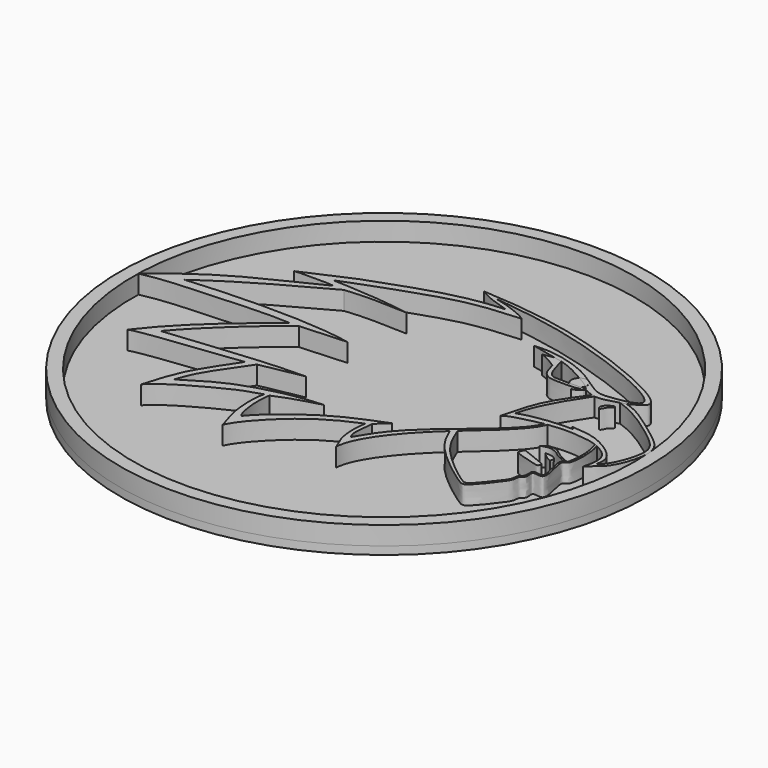
from build123d import *

# Parameters (mm, degrees)
F0_R     = 20
F1_DEPTH = 0.6
F2_R     = 20
F2_R_2   = 19
F3_DEPTH = 1.4
F5_DEPTH = 1.4
F6_DEPTH = 1.4


with BuildPart() as f1:
    # F0 (on Top) → F1 (new body)
    with BuildSketch(Plane.XY):
        Circle(F0_R)
    extrude(amount=-F1_DEPTH)

    # F2 (on Top) → F3 (join)
    with BuildSketch(Plane.XY):
        Circle(F2_R)
        Circle(F2_R_2, mode=Mode.SUBTRACT)
    extrude(amount=F3_DEPTH)


with BuildPart() as f5:
    # F4 (on Top) → F5 (new body)
    with BuildSketch(Plane.XY):
        with BuildLine():
            add(Edge.make_bspline(
                [(-0.4861813504, 11.1744105816), (-0.8512394251, 11.2638310445), (-1.2162974998, 11.3714220446), (-1.5813555744, 11.4608425075)],
                knots=[0, 0, 0, 0, 1.1320114085, 1.1320114085, 1.1320114085, 1.1320114085], degree=3))
            add(Edge.make_bspline(
                [(0.8560517081, 10.4608425075), (0.4573200056, 10.5881941765), (-0.7648135611, 10.9467365684), (-1.4453119288, 11.3807328225), (-1.5813555744, 11.4608425075)],
                knots=[0, 0, 0, 0, 0.579016689, 1, 1, 1, 1], degree=3))
            add(Edge.make_bspline(
                [(0.8560517081, 10.4608425075), (1.347997395, 10.3502387475), (1.8399430819, 10.2214644504), (2.3318887688, 10.1108606905)],
                knots=[0, 0, 0, 0, 1.5167670559, 1.5167670559, 1.5167670559, 1.5167670559], degree=3))
            add(Edge.make_bspline(
                [(-0.4861813504, 11.1744105816), (-0.0018532867, 11.0755696507), (0.8729949517, 10.8262661766), (2.0316981245, 10.3485118598), (2.3318887688, 10.1108606905)],
                knots=[0, 0, 0, 0, 0.493621531, 1, 1, 1, 1], degree=3))
        make_face()
        with BuildLine():
            add(Edge.make_bspline(
                [(-1.5813555744, 11.4608425075), (1.514651197, 11.2793503488), (6.8334553558, 10.6998128091), (16.2828207566, 6.5822660882), (14.74853224, 5.8477105562), (14.0055896595, 5.4608425075)],
                knots=[0, 0, 0, 0, 0.4316285007, 0.8324272833, 1, 1, 1, 1], degree=3))
            add(Edge.make_bspline(
                [(-0.4861813504, 11.1744105816), (-0.8512394251, 11.2638310445), (-1.2162974998, 11.3714220446), (-1.5813555744, 11.4608425075)],
                knots=[0, 0, 0, 0, 1.1320114085, 1.1320114085, 1.1320114085, 1.1320114085], degree=3))
            add(Edge.make_bspline(
                [(10.5331156468, 6.2760727313), (10.9363930891, 6.0023009623), (11.7608523883, 5.4283523122), (12.6827028969, 5.4977681276), (16.7129876566, 6.1384112415), (6.8471463505, 10.2922851198), (1.9949780392, 10.875952097), (-0.4861813504, 11.1744105816)],
                knots=[0.2889714832, 0.2889714832, 0.2889714832, 0.2889714832, 0.356550035, 0.445023231, 0.5537782213, 0.7718242062, 1, 1, 1, 1], degree=3))
            ThreePointArc((10.5331156468, 6.2760727313), (10.5980424704, 6.205178512), (10.6508136936, 6.1248250382))
            add(Edge.make_bspline(
                [(10.6738684154, 6.0779841061), (10.6672489525, 6.0941943415), (10.6595052577, 6.109775343), (10.6508136936, 6.1248250382)],
                knots=[0.5200267079, 0.5200267079, 0.5200267079, 0.5200267079, 0.5950226776, 0.5950226776, 0.5950226776, 0.5950226776], degree=3))
            ThreePointArc((10.6738684154, 6.0779841061), (10.7117232873, 5.9599696048), (10.7245236322, 5.8366952562))
            ThreePointArc((10.7245236322, 5.8366952562), (10.7193245726, 5.7578800215), (10.7038174948, 5.6804306704))
            add(Edge.make_bspline(
                [(10.8788917387, 5.514291408), (10.8202111372, 5.5743074932), (10.7620872809, 5.6292667311), (10.7038174948, 5.6804306704)],
                knots=[0.0457537508, 0.0457537508, 0.0457537508, 0.0457537508, 0.1098862637, 0.1098862637, 0.1098862637, 0.1098862637], degree=3))
            add(Edge.make_bspline(
                [(11.0055896595, 5.3776609224), (10.9629035479, 5.4260836214), (10.9207559585, 5.4714744204), (10.8788917387, 5.514291408)],
                knots=[0, 0, 0, 0, 0.0457537508, 0.0457537508, 0.0457537508, 0.0457537508], degree=3))
            add(Edge.make_bspline(
                [(11.7051415145, 5.0738393329), (11.478102131, 5.1392894421), (11.2418546361, 5.258068017), (11.0055896595, 5.3776609224)],
                knots=[0.7087711743, 0.7087711743, 0.7087711743, 0.7087711743, 1, 1, 1, 1], degree=3))
            add(Edge.make_bspline(
                [(11.9165486953, 5.0284702119), (11.8452559027, 5.038333895), (11.7756426549, 5.0535155139), (11.7051415145, 5.0738393329)],
                knots=[0.6183376821, 0.6183376821, 0.6183376821, 0.6183376821, 0.7087711743, 0.7087711743, 0.7087711743, 0.7087711743], degree=3))
            add(Edge.make_bspline(
                [(13.5997429191, 5.3412596545), (13.1580057928, 5.2100697092), (12.4957655955, 5.0153138893), (12.0665301911, 5.0077195875), (11.9165486953, 5.0284702119)],
                knots=[0.0995715401, 0.0995715401, 0.0995715401, 0.0995715401, 0.4280891318, 0.6183376821, 0.6183376821, 0.6183376821, 0.6183376821], degree=3))
            add(Edge.make_bspline(
                [(14.0055896595, 5.4608425075), (13.8695725155, 5.4215071201), (13.7336305619, 5.3810224715), (13.5997429191, 5.3412596545)],
                knots=[0, 0, 0, 0, 0.0995715401, 0.0995715401, 0.0995715401, 0.0995715401], degree=3))
        make_face()
        with BuildLine():
            add(Edge.make_bspline(
                [(0.8560517081, 10.4608425075), (1.347997395, 10.3502387475), (1.8399430819, 10.2214644504), (2.3318887688, 10.1108606905)],
                knots=[0, 0, 0, 0, 1.5167670559, 1.5167670559, 1.5167670559, 1.5167670559], degree=3))
            add(Edge.make_bspline(
                [(-11.9944103405, 6.4608425075), (-7.4352765712, 8.5330202898), (-8.3438375258, 7.8825665939), (-2.5707737153, 10.3058462526), (0.8560517081, 10.4608425075)],
                knots=[0, 0, 0, 0, 0.454663222, 1, 1, 1, 1], degree=3))
            add(Edge.make_bspline(
                [(-9.437805973, 6.9979857653), (-10.2901514814, 6.812881167), (-11.1420648321, 6.6459471058), (-11.9944103405, 6.4608425075)],
                knots=[0, 0, 0, 0, 2.6124220125, 2.6124220125, 2.6124220125, 2.6124220125], degree=3))
            add(Edge.make_bspline(
                [(2.3318887688, 10.1108606905), (-0.1704881142, 9.9523263052), (-2.4060494059, 9.6797784859), (-8.1382575205, 7.5277293123), (-9.437805973, 6.9979857653)],
                knots=[0, 0, 0, 0, 0.4735027483, 1, 1, 1, 1], degree=3))
        make_face()
        with BuildLine():
            add(Edge.make_bspline(
                [(-9.437805973, 6.9979857653), (-10.2901514814, 6.812881167), (-11.1420648321, 6.6459471058), (-11.9944103405, 6.4608425075)],
                knots=[0, 0, 0, 0, 2.6124220125, 2.6124220125, 2.6124220125, 2.6124220125], degree=3))
            add(Edge.make_bspline(
                [(-8.9944103405, 6.4608425075), (-9.5227345876, 6.5312589572), (-10.5059407944, 6.462516723), (-11.5227462601, 6.5312941655), (-11.9944103405, 6.4608425075)],
                knots=[0, 0, 0, 0, 0.5049792134, 1, 1, 1, 1], degree=3))
            add(Edge.make_bspline(
                [(-8.9944103405, 6.4608425075), (-8.6776053034, 6.6301364597), (-8.397439304, 6.7902582409), (-8.1671202768, 6.9393072683)],
                knots=[0.8832644452, 0.8832644452, 0.8832644452, 0.8832644452, 0.9755031654, 0.9755031654, 0.9755031654, 0.9755031654], degree=3))
            add(Edge.make_bspline(
                [(-9.437805973, 6.9979857653), (-9.0126793763, 6.9801507696), (-8.5877041172, 6.9611772663), (-8.1671202768, 6.9393072683)],
                knots=[0, 0, 0, 0, 0.199815969, 0.199815969, 0.199815969, 0.199815969], degree=3))
        make_face()
        with BuildLine():
            add(Edge.make_bspline(
                [(8.0055896595, -3.7900607299), (8.290317767, -4.4521385807), (8.9844809049, -5.9540217767), (12.3723434925, -8.4515768964), (13.0451164666, -8.7486977353), (14.3514148065, -7.0178963679), (14.8895121762, -6.3201394359), (14.8316541913, -5.6999676159), (15.339054605, -5.5833601899), (14.9418951503, -4.6397911415), (16.5155754804, -5.3697956819), (15.4397338992, -2.7507088417), (15.9484677785, -2.6639513417), (16.2027573046, -2.339614399), (16.3157848864, -0.8692982274), (16.0055896595, 0.1406914093)],
                knots=[0, 0, 0, 0, 0.1137784461, 0.2601902701, 0.3148507936, 0.417422291, 0.4884856376, 0.539189381, 0.5832073247, 0.6383062782, 0.7002794606, 0.8033644458, 0.8434914934, 0.8846524249, 1, 1, 1, 1], degree=3))
            add(Edge.make_bspline(
                [(16.0055896595, 0.1406914093), (15.936859435, 0.1718639514), (15.8688960906, 0.2002961396), (15.8029496035, 0.2260058139)],
                knots=[0.4452740587, 0.4452740587, 0.4452740587, 0.4452740587, 0.4779418896, 0.4779418896, 0.4779418896, 0.4779418896], degree=3))
            add(Edge.make_bspline(
                [(15.8029496035, 0.2260058139), (16.2006936994, -0.9693456093), (15.9668899378, -2.2166192794), (15.92795558, -2.5949034419), (15.2159733402, -2.5941041989), (16.3932154949, -5.2814039939), (14.8734115826, -4.438489823), (15.1842299283, -5.5488731457), (14.6978233661, -5.6306795332), (14.7380276879, -6.2892111084), (14.2456086984, -6.8848450801), (13.0376296594, -8.4664264452), (12.4637437687, -8.3038412893), (9.1357052886, -5.7276571911), (8.6434670243, -4.1571202739), (8.3486537341, -3.4801096134)],
                knots=[0, 0, 0, 0, 0.1170783241, 0.1538590408, 0.1984892764, 0.3021938664, 0.3631383845, 0.4243811494, 0.4678027754, 0.5205636841, 0.5883717685, 0.6881215272, 0.7381813319, 0.8845935619, 1, 1, 1, 1], degree=3))
            add(Edge.make_bspline(
                [(8.0055896595, -3.7900607299), (8.1183412502, -3.6872860039), (8.2326324706, -3.5841350133), (8.3486537341, -3.4801096134)],
                knots=[0.5563520178, 0.5563520178, 0.5563520178, 0.5563520178, 0.5913081958, 0.5913081958, 0.5913081958, 0.5913081958], degree=3))
        make_face()
        with BuildLine():
            add(Edge.make_bspline(
                [(-8.9944103405, 6.4608425075), (-8.7216751352, 6.456489241), (-8.4493720874, 6.4339654374), (-8.1766368821, 6.4296121709)],
                knots=[0, 0, 0, 0, 0.8183695761, 0.8183695761, 0.8183695761, 0.8183695761], degree=3))
            add(Edge.make_bspline(
                [(-18.9944103405, 0.4608425075), (-17.5819190405, 1.6336166373), (-14.9380365277, 3.719038189), (-10.3751922712, 5.7229816691), (-8.9944103405, 6.4608425075)],
                knots=[0, 0, 0, 0, 0.4812457167, 0.8832644452, 0.8832644452, 0.8832644452, 0.8832644452], degree=3))
            add(Edge.make_bspline(
                [(-16.3652878255, 1.5516962158), (-17.2418060497, 1.1820214673), (-18.1178921163, 0.8305172559), (-18.9944103405, 0.4608425075)],
                knots=[0, 0, 0, 0, 2.8464446265, 2.8464446265, 2.8464446265, 2.8464446265], degree=3))
            add(Edge.make_bspline(
                [(-8.1766368821, 6.4296121709), (-10.0553413983, 5.4250495729), (-13.461796709, 3.559962101), (-15.4947216945, 2.1565062864), (-16.3652878255, 1.5516962158)],
                knots=[0, 0, 0, 0, 0.571381465, 1, 1, 1, 1], degree=3))
        make_face()
        with BuildLine():
            add(Edge.make_bspline(
                [(-8.9944103405, 6.4608425075), (-8.6776053034, 6.6301364597), (-8.397439304, 6.7902582409), (-8.1671202768, 6.9393072683)],
                knots=[0.8832644452, 0.8832644452, 0.8832644452, 0.8832644452, 0.9755031654, 0.9755031654, 0.9755031654, 0.9755031654], degree=3))
            add(Edge.make_bspline(
                [(-8.9944103405, 6.4608425075), (-8.7216751352, 6.456489241), (-8.4493720874, 6.4339654374), (-8.1766368821, 6.4296121709)],
                knots=[0, 0, 0, 0, 0.8183695761, 0.8183695761, 0.8183695761, 0.8183695761], degree=3))
            add(Edge.make_bspline(
                [(-3.4766462632, 6.4608425075), (-4.6195223532, 6.4761082239), (-6.0056012046, 6.5942768078), (-7.709692655, 6.4793701805), (-8.1766368821, 6.4296121709)],
                knots=[0, 0, 0, 0, 0.5412673538, 1, 1, 1, 1], degree=3))
            add(Edge.make_bspline(
                [(-8.1671202768, 6.9393072683), (-7.4883861721, 6.9040136786), (-5.8324939664, 6.79771411), (-4.3567601819, 6.5994669238), (-3.4766462632, 6.4608425075)],
                knots=[0.199815969, 0.199815969, 0.199815969, 0.199815969, 0.5222770334, 1, 1, 1, 1], degree=3))
        make_face()
        with BuildLine():
            add(Edge.make_bspline(
                [(4.0055896595, -9.5391574925), (4.0640229048, -8.4050470974), (5.6258918331, -6.0675921748), (7.2579217171, -4.4715710079), (8.0055896595, -3.7900607299)],
                knots=[0, 0, 0, 0, 0.3245538369, 0.5563520178, 0.5563520178, 0.5563520178, 0.5563520178], degree=3))
            add(Edge.make_bspline(
                [(8.0055896595, -3.7900607299), (8.1183412502, -3.6872860039), (8.2326324706, -3.5841350133), (8.3486537341, -3.4801096134)],
                knots=[0.5563520178, 0.5563520178, 0.5563520178, 0.5563520178, 0.5913081958, 0.5913081958, 0.5913081958, 0.5913081958], degree=3))
            add(Edge.make_bspline(
                [(8.3486537341, -3.4801096134), (8.5877905191, -3.2656980569), (9.9859491551, -2.0284086781), (11.6742389457, -0.5312455851), (12.0055896595, 0.4608425075)],
                knots=[0.5913081958, 0.5913081958, 0.5913081958, 0.5913081958, 0.6633579887, 1, 1, 1, 1], degree=3))
            add(Edge.make_bspline(
                [(11.8052601549, 0.4324009459), (11.8704997149, 0.4414805342), (11.9403500995, 0.4517629192), (12.0055896595, 0.4608425075)],
                knots=[0, 0, 0, 0, 0.2023384117, 0.2023384117, 0.2023384117, 0.2023384117], degree=3))
            add(Edge.make_bspline(
                [(3.9102742448, -8.0432752147), (4.3585507686, -7.225709157), (5.503324856, -5.5090435402), (8.5702876807, -2.9413221208), (11.3297734442, -0.6915840851), (11.8052601549, 0.4324009459)],
                knots=[0, 0, 0, 0, 0.2886820024, 0.6363748963, 1, 1, 1, 1], degree=3))
            add(Edge.make_bspline(
                [(3.8548011798, -5.9568551369), (3.772172657, -6.5835202766), (3.644234835, -7.5538168559), (3.8406969894, -7.9152672279), (3.9102742448, -8.0432752147)],
                knots=[0, 0, 0, 0, 0.6458490662, 1, 1, 1, 1], degree=3))
            add(Edge.make_bspline(
                [(3.5055896595, -6.1596883461), (3.6221375521, -6.0920772764), (3.7382532872, -6.0244662066), (3.8548011798, -5.9568551369)],
                knots=[0, 0, 0, 0, 0.4038440252, 0.4038440252, 0.4038440252, 0.4038440252], degree=3))
            add(Edge.make_bspline(
                [(3.5055896595, -6.1596883461), (3.3600590635, -6.9084815459), (3.4432477493, -8.5297381785), (3.7729906459, -8.9020562877), (4.0055896595, -9.5391574925)],
                knots=[0, 0, 0, 0, 0.5658292742, 1, 1, 1, 1], degree=3))
        make_face()
        with BuildLine():
            add(Edge.make_bspline(
                [(-16.3652878255, 1.5516962158), (-17.2418060497, 1.1820214673), (-18.1178921163, 0.8305172559), (-18.9944103405, 0.4608425075)],
                knots=[0, 0, 0, 0, 2.8464446265, 2.8464446265, 2.8464446265, 2.8464446265], degree=3))
            add(Edge.make_bspline(
                [(-7.9944103405, 1.1069288947), (-9.4193134786, 1.237536743), (-13.8743454501, 0.9399078326), (-17.3496462389, 0.824787051), (-18.9944103405, 0.4608425075)],
                knots=[0, 0, 0, 0, 0.5087005402, 1, 1, 1, 1], degree=3))
            add(Edge.make_bspline(
                [(-7.9944103405, 1.1069288947), (-7.7784326722, 1.118545444), (-7.5628871615, 1.1301619933), (-7.3469094932, 1.1417785427)],
                knots=[0, 0, 0, 0, 0.6484380041, 0.6484380041, 0.6484380041, 0.6484380041], degree=3))
            add(Edge.make_bspline(
                [(-3.8513934705, 1.3500220375), (-5.0165654781, 1.2806075392), (-6.1817374857, 1.2111930409), (-7.3469094932, 1.1417785427)],
                knots=[0, 0, 0, 0, 3.501713526, 3.501713526, 3.501713526, 3.501713526], degree=3))
            add(Edge.make_bspline(
                [(-16.3652878255, 1.5516962158), (-15.565707993, 1.6230606445), (-13.3888340962, 1.8009877733), (-6.9601712748, 1.95987802), (-3.8513934705, 1.3500220375)],
                knots=[0, 0, 0, 0, 0.3529099079, 1, 1, 1, 1], degree=3))
        make_face()
        with BuildLine():
            add(Edge.make_bspline(
                [(11.8052601549, 0.4324009459), (11.8704997149, 0.4414805342), (11.9403500995, 0.4517629192), (12.0055896595, 0.4608425075)],
                knots=[0, 0, 0, 0, 0.2023384117, 0.2023384117, 0.2023384117, 0.2023384117], degree=3))
            add(Edge.make_bspline(
                [(12.0055896595, 0.4608425075), (11.9332310752, 0.4510848131), (11.8667309035, 0.4416234795), (11.8052601549, 0.4324009459)],
                knots=[0, 0, 0, 0, 0.0453625168, 0.0453625168, 0.0453625168, 0.0453625168], degree=3))
        make_face()
        with BuildLine():
            add(Edge.make_bspline(
                [(11.0055896595, 5.3776609224), (10.9768566842, 5.3499833826), (10.9481051428, 5.3223087447), (10.9193240765, 5.2950871694)],
                knots=[0, 0, 0, 0, 0.1162457919, 0.1162457919, 0.1162457919, 0.1162457919], degree=3))
            add(Edge.make_bspline(
                [(11.0055896595, 5.3776609224), (10.9629035479, 5.4260836214), (10.9207559585, 5.4714744204), (10.8788917387, 5.514291408)],
                knots=[0, 0, 0, 0, 0.0457537508, 0.0457537508, 0.0457537508, 0.0457537508], degree=3))
            add(Edge.make_bspline(
                [(10.7126522699, 5.2433540713), (10.7778732235, 5.3274456432), (10.828419646, 5.4209023466), (10.8788917387, 5.514291408)],
                knots=[0.6310392789, 0.6310392789, 0.6310392789, 0.6310392789, 1, 1, 1, 1], degree=3))
            add(Edge.make_bspline(
                [(10.7126522759, 5.24335406), (10.7999302605, 5.2588050266), (10.8708150905, 5.2773339919), (10.912349001, 5.291994101), (10.9193240765, 5.2950871694)],
                knots=[0.8539309447, 0.8539309447, 0.8539309447, 0.8539309447, 0.9271004176, 0.9428592974, 0.9428592974, 0.9428592974, 0.9428592974], degree=3))
        make_face()
        with BuildLine():
            add(Edge.make_bspline(
                [(-7.9944103405, 1.1069288947), (-7.7784326722, 1.118545444), (-7.5628871615, 1.1301619933), (-7.3469094932, 1.1417785427)],
                knots=[0, 0, 0, 0, 0.6484380041, 0.6484380041, 0.6484380041, 0.6484380041], degree=3))
            add(Edge.make_bspline(
                [(-14.9944103405, -5.5391574925), (-13.7942935133, -3.9556998013), (-11.3643048238, -1.5615426011), (-8.5238665029, 0.7570548369), (-7.9944103405, 1.1069288947)],
                knots=[0, 0, 0, 0, 0.5500986234, 1, 1, 1, 1], degree=3))
            add(Edge.make_bspline(
                [(-13.3645571768, -4.4584060088), (-13.9079856172, -4.8247133491), (-14.4509819001, -5.1728501522), (-14.9944103405, -5.5391574925)],
                knots=[0, 0, 0, 0, 1.9556188547, 1.9556188547, 1.9556188547, 1.9556188547], degree=3))
            add(Edge.make_bspline(
                [(-7.3469094932, 1.1417785427), (-8.4448163694, 0.338849624), (-10.428148874, -1.3877723247), (-12.459579288, -3.3913620914), (-13.3645571768, -4.4584060088)],
                knots=[0, 0, 0, 0, 0.4931522989, 1, 1, 1, 1], degree=3))
        make_face()
        with BuildLine():
            add(Edge.make_bspline(
                [(3.5055896595, -6.1596883461), (1.5482186348, -6.9707707492), (-0.6694731698, -8.506315502), (-2.5806236884, -10.6681760377), (-2.9944103405, -11.5391574925)],
                knots=[0, 0, 0, 0, 0.5459799602, 1, 1, 1, 1], degree=3))
            add(Edge.make_bspline(
                [(3.5055896595, -6.1596883461), (3.6221375521, -6.0920772764), (3.7382532872, -6.0244662066), (3.8548011798, -5.9568551369)],
                knots=[0, 0, 0, 0, 0.4038440252, 0.4038440252, 0.4038440252, 0.4038440252], degree=3))
            add(Edge.make_bspline(
                [(4.7053410672, -5.1438389346), (4.1925152764, -5.5566010997), (4.1383144756, -5.6858497361), (3.8548011798, -5.9568551369)],
                knots=[0, 0, 0, 0, 1.1766109999, 1.1766109999, 1.1766109999, 1.1766109999], degree=3))
            add(Edge.make_bspline(
                [(-2.8363403399, -9.9698845297), (-2.2336716839, -9.1870877606), (0.8173735421, -6.6037034172), (3.4794779633, -5.6316827497), (4.7053410672, -5.1438389346)],
                knots=[0, 0, 0, 0, 0.5101080536, 1, 1, 1, 1], degree=3))
            add(Edge.make_bspline(
                [(-2.8363403399, -9.9698845297), (-2.8891743926, -10.499032363), (-2.9415762878, -11.0100096592), (-2.9944103405, -11.5391574925)],
                knots=[0, 0, 0, 0, 1.5772139224, 1.5772139224, 1.5772139224, 1.5772139224], degree=3))
        make_face()
        with BuildLine():
            add(Edge.make_bspline(
                [(10.7126522699, 5.2433540713), (10.7778732235, 5.3274456432), (10.828419646, 5.4209023466), (10.8788917387, 5.514291408)],
                knots=[0.6310392789, 0.6310392789, 0.6310392789, 0.6310392789, 1, 1, 1, 1], degree=3))
            add(Edge.make_bspline(
                [(10.5876969687, 5.4552893565), (10.7120407688, 5.4688463016), (10.8133734046, 5.4879357632), (10.8788917387, 5.514291408)],
                knots=[0.9288848526, 0.9288848526, 0.9288848526, 0.9288848526, 1, 1, 1, 1], degree=3))
            ThreePointArc((10.5876969687, 5.4552893565), (10.1438280298, 5.2370058864), (9.686839216, 5.4262901493))
            add(Edge.make_bspline(
                [(7.5754439722, 7.3132768172), (7.7364737299, 6.7638616103), (7.9648004439, 5.8004228314), (8.4151602101, 5.4504426739), (8.6409937872, 5.4554326027), (9.3331000431, 5.4294527687), (9.686839216, 5.4262901493)],
                knots=[0, 0, 0, 0, 0.3160564432, 0.4833699083, 0.6372331155, 0.7893674455, 0.7893674455, 0.7893674455, 0.7893674455], degree=3))
            add(Edge.make_bspline(
                [(7.0055896595, 7.4340827679), (7.1942274201, 7.3945596872), (7.3868062116, 7.3527998979), (7.5754439722, 7.3132768172)],
                knots=[0, 0, 0, 0, 0.5825186824, 0.5825186824, 0.5825186824, 0.5825186824], degree=3))
            add(Edge.make_bspline(
                [(7.0055896595, 7.4340827679), (7.2380322538, 7.1423215901), (7.3789222386, 6.8507832218), (7.476943944, 6.5867935747)],
                knots=[0, 0, 0, 0, 0.1155563183, 0.1155563183, 0.1155563183, 0.1155563183], degree=3))
            add(Edge.make_bspline(
                [(7.476943944, 6.5867935747), (7.5999064538, 6.2556339662), (7.7042415865, 5.7146182621), (8.0113414198, 5.4199653425), (8.4127104593, 5.1092583158), (10.1484899112, 5.1607212843), (10.6451011692, 5.2313953753), (10.7126522759, 5.24335406)],
                knots=[0.1155563183, 0.1155563183, 0.1155563183, 0.1155563183, 0.2605149769, 0.3880464278, 0.5226573434, 0.7972994941, 0.8539309447, 0.8539309447, 0.8539309447, 0.8539309447], degree=3))
        make_face()
        with BuildLine():
            add(Edge.make_bspline(
                [(10.9193240765, 5.2950871694), (10.8136287363, 5.1951188902), (10.5939974651, 5.0008170496), (10.370333691, 4.9282497859), (10.2546671405, 4.8907813616)],
                knots=[0.1162457919, 0.1162457919, 0.1162457919, 0.1162457919, 0.5431458381, 1, 1, 1, 1], degree=3))
            add(Edge.make_bspline(
                [(10.7126522759, 5.24335406), (10.7999302605, 5.2588050266), (10.8708150905, 5.2773339919), (10.912349001, 5.291994101), (10.9193240765, 5.2950871694)],
                knots=[0.8539309447, 0.8539309447, 0.8539309447, 0.8539309447, 0.9271004176, 0.9428592974, 0.9428592974, 0.9428592974, 0.9428592974], degree=3))
            add(Edge.make_bspline(
                [(10.2546671405, 4.8907813616), (10.3986650181, 4.9756816362), (10.5737070223, 5.0788817123), (10.6928685377, 5.2178462391), (10.7126522699, 5.2433540713)],
                knots=[0, 0, 0, 0, 0.5191209503, 0.6310392789, 0.6310392789, 0.6310392789, 0.6310392789], degree=3))
        make_face()
        with BuildLine():
            add(Edge.make_bspline(
                [(-13.3645571768, -4.4584060088), (-13.9079856172, -4.8247133491), (-14.4509819001, -5.1728501522), (-14.9944103405, -5.5391574925)],
                knots=[0, 0, 0, 0, 1.9556188547, 1.9556188547, 1.9556188547, 1.9556188547], degree=3))
            add(Edge.make_bspline(
                [(-6.9944103405, -4.4383769855), (-8.0951718683, -4.5501379279), (-8.9273283999, -4.7239324162), (-14.1716016041, -5.2542345674), (-14.9944103405, -5.5391574925)],
                knots=[0, 0, 0, 0, 0.4007344326, 1, 1, 1, 1], degree=3))
            add(Edge.make_bspline(
                [(-6.9944103405, -4.4383769855), (-6.7415432408, -4.3755271472), (-6.4891082987, -4.3126773089), (-6.2362411991, -4.2498274706)],
                knots=[0, 0, 0, 0, 0.7812626745, 0.7812626745, 0.7812626745, 0.7812626745], degree=3))
            add(Edge.make_bspline(
                [(-3.0233417638, -3.6399713717), (-4.0005971612, -3.8386157244), (-5.4580878496, -4.0878689765), (-6.0480198511, -4.2227470447), (-6.2362411991, -4.2498274706)],
                knots=[0, 0, 0, 0, 0.6546808205, 1, 1, 1, 1], degree=3))
            add(Edge.make_bspline(
                [(-13.3645571768, -4.4584060088), (-12.0681423322, -4.3195819823), (-9.1183843322, -4.0484323098), (-5.700757727, -3.6697206087), (-3.0233417638, -3.6399713717)],
                knots=[0, 0, 0, 0, 0.443130057, 1, 1, 1, 1], degree=3))
        make_face()
        with BuildLine():
            add(Edge.make_bspline(
                [(7.0055896595, 7.4340827679), (7.2380322538, 7.1423215901), (7.3789222386, 6.8507832218), (7.476943944, 6.5867935747)],
                knots=[0, 0, 0, 0, 0.1155563183, 0.1155563183, 0.1155563183, 0.1155563183], degree=3))
            add(Edge.make_bspline(
                [(7.0055896595, 7.4340827679), (6.8483246088, 7.4388027019), (6.526745131, 7.363842235), (6.3055163314, 7.3433438763), (6.1365221627, 7.2932951152)],
                knots=[0, 0, 0, 0, 0.5138358463, 1, 1, 1, 1], degree=3))
            add(Edge.make_bspline(
                [(7.476943944, 6.5867935747), (7.2756173457, 6.7262404804), (6.8580098112, 6.9870822905), (6.3467008971, 7.2284280765), (6.1365221627, 7.2932951152)],
                knots=[0, 0, 0, 0, 0.4974955898, 1, 1, 1, 1], degree=3))
        make_face()
        with BuildLine():
            add(Edge.make_bspline(
                [(-2.9944103405, -11.5391574925), (-3.3684727764, -10.2999222363), (-3.5596399169, -9.9490778974), (-3.7298861371, -7.5312945942), (-3.4944103405, -6.9626686163)],
                knots=[0, 0, 0, 0, 0.4778739361, 1, 1, 1, 1], degree=3))
            add(Edge.make_bspline(
                [(-2.8363403399, -9.9698845297), (-2.8891743926, -10.499032363), (-2.9415762878, -11.0100096592), (-2.9944103405, -11.5391574925)],
                knots=[0, 0, 0, 0, 1.5772139224, 1.5772139224, 1.5772139224, 1.5772139224], degree=3))
            add(Edge.make_bspline(
                [(-3.1803087331, -6.8991845474), (-3.3214866512, -7.8015294341), (-3.1952766606, -9.0527440799), (-3.0059898672, -9.7746249419), (-2.8363403399, -9.9698845297)],
                knots=[0, 0, 0, 0, 0.6138067856, 1, 1, 1, 1], degree=3))
            add(Edge.make_bspline(
                [(-3.1803087331, -6.8991845474), (-3.2851533214, -6.9203459037), (-3.3895657522, -6.94150726), (-3.4944103405, -6.9626686163)],
                knots=[0, 0, 0, 0, 0.3204528776, 0.3204528776, 0.3204528776, 0.3204528776], degree=3))
        make_face()
        with BuildLine():
            add(Edge.make_bspline(
                [(-6.9944103405, -4.4383769855), (-6.7415432408, -4.3755271472), (-6.4891082987, -4.3126773089), (-6.2362411991, -4.2498274706)],
                knots=[0, 0, 0, 0, 0.7812626745, 0.7812626745, 0.7812626745, 0.7812626745], degree=3))
            add(Edge.make_bspline(
                [(-9.9944103405, -10.5391574925), (-9.3742412685, -8.2597849546), (-8.566524745, -6.8345184853), (-7.3733651334, -4.9659464193), (-6.9944103405, -4.4383769855)],
                knots=[0, 0, 0, 0, 0.5731045047, 1, 1, 1, 1], degree=3))
            add(Edge.make_bspline(
                [(-8.8671809062, -8.8074477389), (-9.2430681035, -9.3907411692), (-9.6185231432, -9.9558640623), (-9.9944103405, -10.5391574925)],
                knots=[0, 0, 0, 0, 2.0662683437, 2.0662683437, 2.0662683437, 2.0662683437], degree=3))
            add(Edge.make_bspline(
                [(-6.2362411991, -4.2498274706), (-6.8336737535, -5.1070575407), (-8.3886130268, -7.3405128695), (-8.6195366457, -8.135269396), (-8.8671809062, -8.8074477389)],
                knots=[0, 0, 0, 0, 0.5932918079, 1, 1, 1, 1], degree=3))
        make_face()
        with BuildLine():
            add(Edge.make_bspline(
                [(-3.4944103405, -6.9626686163), (-4.6174455846, -7.3435130285), (-4.6436947556, -7.2200525115), (-9.3684580041, -9.6523935135), (-9.9944103405, -10.5391574925)],
                knots=[0, 0, 0, 0, 0.3682839224, 1, 1, 1, 1], degree=3))
            add(Edge.make_bspline(
                [(-3.1803087331, -6.8991845474), (-3.2851533214, -6.9203459037), (-3.3895657522, -6.94150726), (-3.4944103405, -6.9626686163)],
                knots=[0, 0, 0, 0, 0.3204528776, 0.3204528776, 0.3204528776, 0.3204528776], degree=3))
            add(Edge.make_bspline(
                [(0.0970787078, -5.8130566031), (-0.4660853592, -5.9673427604), (-1.0216870143, -6.1379982253), (-2.0933459666, -6.4298141805), (-3.1803087331, -6.8991845474)],
                knots=[0, 0, 0, 0, 0.4152091703, 1, 1, 1, 1], degree=3))
            add(Edge.make_bspline(
                [(-8.8671809062, -8.8074477389), (-7.8682395965, -8.1962507687), (-5.7447688574, -6.7453350294), (-1.6718116822, -5.8749676682), (0.0970787078, -5.8130566031)],
                knots=[0, 0, 0, 0, 0.4445935625, 1, 1, 1, 1], degree=3))
            add(Edge.make_bspline(
                [(-8.8671809062, -8.8074477389), (-9.2430681035, -9.3907411692), (-9.6185231432, -9.9558640623), (-9.9944103405, -10.5391574925)],
                knots=[0, 0, 0, 0, 2.0662683437, 2.0662683437, 2.0662683437, 2.0662683437], degree=3))
        make_face()
    extrude(amount=F5_DEPTH)


with BuildPart() as f5b:
    # F4 (on Top) → F5, piece 2 (new body)
    with BuildSketch(Plane.XY):
        with BuildLine():
            ThreePointArc((9.753270105, 6.308045252), (10.0564087743, 6.4328163564), (10.3798798954, 6.379643853))
            add(Edge.make_bspline(
                [(5.0704041496, 7.8671742231), (5.4646223846, 7.8945418861), (6.4589528684, 7.9635709143), (8.7973510038, 7.4072181903), (10.0609980807, 6.5939097333), (10.3798798954, 6.379643853)],
                knots=[0, 0, 0, 0, 0.0906207262, 0.2285712393, 0.2805322177, 0.2805322177, 0.2805322177, 0.2805322177], degree=3))
            add(Edge.make_bspline(
                [(7.0055896595, 7.4340827679), (6.6557129965, 7.5247258548), (5.975924053, 7.6601243944), (5.3660957164, 7.803766372), (5.0704041496, 7.8671742231)],
                knots=[0, 0, 0, 0, 0.5174156898, 1, 1, 1, 1], degree=3))
            add(Edge.make_bspline(
                [(7.5754439722, 7.3132768172), (7.3900309525, 7.3642812964), (7.1997902119, 7.4056356612), (7.0055896595, 7.4340827679)],
                knots=[0.8977080162, 0.8977080162, 0.8977080162, 0.8977080162, 1, 1, 1, 1], degree=3))
            add(Edge.make_bspline(
                [(9.753270105, 6.308045252), (9.1880367304, 6.6345998901), (8.4334284517, 7.0772575151), (7.5754439722, 7.3132768172)],
                knots=[0.4243597333, 0.4243597333, 0.4243597333, 0.4243597333, 0.8977080162, 0.8977080162, 0.8977080162, 0.8977080162], degree=3))
        make_face()
    extrude(amount=F5_DEPTH)


with BuildPart() as f5c:
    # F4 (on Top) → F5, piece 3 (new body)
    with BuildSketch(Plane.XY):
        with BuildLine():
            ThreePointArc((10.5876969687, 5.4552893565), (10.657774622, 5.5616618366), (10.7038174948, 5.6804306704))
            add(Edge.make_bspline(
                [(10.7038174948, 5.6804306704), (10.4254151456, 5.9248825869), (10.1362706847, 6.0868484611), (9.7628947949, 6.3024847397), (9.753270105, 6.308045252)],
                knots=[0.1098862637, 0.1098862637, 0.1098862637, 0.1098862637, 0.4162996458, 0.4243597333, 0.4243597333, 0.4243597333, 0.4243597333], degree=3))
            ThreePointArc((9.753270105, 6.308045252), (9.5262192244, 5.8817711436), (9.686839216, 5.4262901493))
            add(Edge.make_bspline(
                [(9.686839216, 5.4262901493), (10.011241816, 5.4233898147), (10.3437528131, 5.428692634), (10.5876969687, 5.4552893565)],
                knots=[0.7893674455, 0.7893674455, 0.7893674455, 0.7893674455, 0.9288848526, 0.9288848526, 0.9288848526, 0.9288848526], degree=3))
        make_face()
    extrude(amount=F5_DEPTH)


with BuildPart() as f5d:
    # F4 (on Top) → F5, piece 4 (new body)
    with BuildSketch(Plane.XY):
        with BuildLine():
            add(Edge.make_bspline(
                [(15.0166591629, -3.0328873545), (14.8289271144, -2.977658953), (14.579419011, -2.8200348556), (14.2519401221, -2.5694584846), (14.1962645575, -2.4386267178)],
                knots=[0, 0, 0, 0, 0.5013763221, 1, 1, 1, 1], degree=3))
            add(Edge.make_bspline(
                [(14.1962645575, -2.4386267178), (14.3243505563, -2.474091232), (14.5566133771, -2.4338478117), (14.9673135163, -2.5798806066), (15.0577574353, -2.7866188023), (15.0279821445, -2.9602306806), (15.0166591629, -3.0328873545)],
                knots=[0, 0, 0, 0, 0.2800515295, 0.5692061441, 0.7754675717, 1, 1, 1, 1], degree=3))
        make_face()
    extrude(amount=F5_DEPTH)


with BuildPart() as f5e:
    # F4 (on Top) → F5, piece 5 (new body)
    with BuildSketch(Plane.XY):
        with BuildLine():
            add(Edge.make_bspline(
                [(15.6757831573, -2.5491658598), (15.5804967169, -2.5348730203), (15.5097852205, -2.539949552), (14.8815367571, -2.2217926339), (14.7052041272, -2.0078864536), (14.0075978186, -1.6873081937), (13.5486286244, -1.8547309471), (13.3373988792, -1.951631275)],
                knots=[0, 0, 0, 0, 0.127602772, 0.3560877522, 0.518700647, 0.7575961092, 1, 1, 1, 1], degree=3))
            add(Edge.make_bspline(
                [(15.6757831573, -2.5491658598), (15.7188904445, -2.5599426816), (15.8044281877, -2.5252249278), (15.846827513, -2.5363364068), (15.8858858049, -2.4896676186)],
                knots=[0, 0, 0, 0, 0.5236012195, 1, 1, 1, 1], degree=3))
            add(Edge.make_bspline(
                [(13.3373988792, -1.951631275), (13.4808437724, -1.7994007422), (13.8393374483, -1.5966043948), (14.3073780775, -1.6344663908), (14.5813395519, -1.744710437), (15.0536914932, -2.1938165325), (15.5297726614, -2.3750418621), (15.7848894108, -2.518583576), (15.8858858049, -2.4896676186)],
                knots=[0, 0, 0, 0, 0.1901490461, 0.3512654216, 0.4825183776, 0.6763356784, 0.8558883201, 1, 1, 1, 1], degree=3))
        make_face()
    extrude(amount=F5_DEPTH)


with BuildPart() as f5f:
    # F4 (on Top) → F5, piece 6 (new body)
    with BuildSketch(Plane.XY):
        with BuildLine():
            add(Edge.make_bspline(
                [(14.5235862583, -3.9308825508), (14.1481318445, -3.8389207533), (12.9666371586, -3.5181886782), (12.8219016087, -3.3438601917), (12.8980182445, -3.2009991292), (12.954743021, -2.9864790438), (13.0803828469, -2.9221494616), (13.2149860237, -3.0091750226), (14.6793113647, -3.5718388249), (14.8619141768, -3.6418550318), (14.9184337185, -3.7602676441), (14.8432189314, -3.9376521646), (14.7760719976, -3.9870009769), (14.6749975062, -3.9679684126), (14.5235862583, -3.9308825508)],
                knots=[0, 0, 0, 0, 0.1965348484, 0.2609912403, 0.318742608, 0.3915515062, 0.4415614166, 0.5030473002, 0.6964541821, 0.7664396, 0.8159812122, 0.8818077175, 0.9207424775, 1, 1, 1, 1], degree=3))
        make_face()
    extrude(amount=F5_DEPTH)


with BuildPart() as f5g:
    # F4 (on Top) → F5, piece 7 (new body)
    with BuildSketch(Plane.XY):
        with BuildLine():
            add(Edge.make_bspline(
                [(13.6758415028, 4.7596092336), (13.5967514361, 4.7994285712), (13.1085024743, 4.5628672925), (12.9487815042, 4.1578801595), (13.2075850142, 3.8624631227), (13.3992486383, 4.5425383048), (13.7117965258, 4.612714891), (13.7098446564, 4.7424897253), (13.6758415028, 4.7596092336)],
                knots=[0, 0, 0, 0, 0.2147215115, 0.4045126008, 0.5322187037, 0.7487907564, 0.907684886, 1, 1, 1, 1], degree=3))
        make_face()
    extrude(amount=F5_DEPTH)


with BuildPart() as f6:
    # F4 (on Top) → F6 (new body)
    with BuildSketch(Plane.XY):
        with BuildLine():
            ThreePointArc((10.6738684154, 6.0779841061), (10.6628507613, 6.1016554457), (10.6508136936, 6.1248250382))
            add(Edge.make_bspline(
                [(10.6508136936, 6.1248250382), (10.6123350392, 6.1914519435), (10.5552786698, 6.2476655358), (10.4949474483, 6.3019629078)],
                knots=[0.5950226776, 0.5950226776, 0.5950226776, 0.5950226776, 0.9270393287, 0.9270393287, 0.9270393287, 0.9270393287], degree=3))
            add(Edge.make_bspline(
                [(10.3798798954, 6.379643853), (10.4186342348, 6.3536036957), (10.4569918517, 6.327685545), (10.4949474483, 6.3019629078)],
                knots=[0.2805322177, 0.2805322177, 0.2805322177, 0.2805322177, 0.2868471385, 0.2868471385, 0.2868471385, 0.2868471385], degree=3))
            ThreePointArc((10.3798798954, 6.379643853), (10.0564087743, 6.4328163564), (9.753270105, 6.308045252))
            add(Edge.make_bspline(
                [(10.7038174948, 5.6804306704), (10.4254151456, 5.9248825869), (10.1362706847, 6.0868484611), (9.7628947949, 6.3024847397), (9.753270105, 6.308045252)],
                knots=[0.1098862637, 0.1098862637, 0.1098862637, 0.1098862637, 0.4162996458, 0.4243597333, 0.4243597333, 0.4243597333, 0.4243597333], degree=3))
            add(Edge.make_bspline(
                [(10.7038174948, 5.6804306704), (10.7116135077, 5.8229242202), (10.7197681819, 5.965581328), (10.6738684154, 6.0779841061)],
                knots=[0, 0, 0, 0, 0.5200267079, 0.5200267079, 0.5200267079, 0.5200267079], degree=3))
        make_face()
    extrude(amount=F6_DEPTH)


with BuildPart() as f6b:
    # F4 (on Top) → F6, piece 2 (new body)
    with BuildSketch(Plane.XY):
        with BuildLine():
            ThreePointArc((9.686839216, 5.4262901493), (10.1438280298, 5.2370058864), (10.5876969687, 5.4552893565))
            add(Edge.make_bspline(
                [(9.686839216, 5.4262901493), (10.011241816, 5.4233898147), (10.3437528131, 5.428692634), (10.5876969687, 5.4552893565)],
                knots=[0.7893674455, 0.7893674455, 0.7893674455, 0.7893674455, 0.9288848526, 0.9288848526, 0.9288848526, 0.9288848526], degree=3))
        make_face()
    extrude(amount=F6_DEPTH)


with BuildPart() as f6c:
    # F4 (on Top) → F6, piece 3 (new body)
    with BuildSketch(Plane.XY):
        with BuildLine():
            add(Edge.make_bspline(
                [(14.0055896595, 5.4608425075), (14.9418430478, 5.1981285129), (16.4001355545, 4.1423648305), (18.0839441101, 2.9416301344), (19.3501189861, 1.6467818438), (18.3202160057, -1.5540488014), (17.475680135, -1.9312547477), (17.0011911541, -2.3996017408)],
                knots=[0, 0, 0, 0, 0.2265953928, 0.4218314589, 0.5945152784, 0.8258761034, 1, 1, 1, 1], degree=3))
            add(Edge.make_bspline(
                [(13.5997429191, 5.3412596545), (13.7334234365, 5.3799916911), (13.8719091421, 5.4221104709), (14.0055896595, 5.4608425075)],
                knots=[0, 0, 0, 0, 0.4230976665, 0.4230976665, 0.4230976665, 0.4230976665], degree=3))
            add(Edge.make_bspline(
                [(17.3990372568, -1.7081559636), (17.5657166254, -1.576362261), (18.0497213335, -1.1867824848), (19.0506363966, 1.4735592991), (18.0181124579, 2.6701819874), (16.0780590799, 4.1293659644), (14.6025343579, 5.0011555878), (13.5997429191, 5.3412596545)],
                knots=[0, 0, 0, 0, 0.1290289728, 0.361910461, 0.5345527105, 0.7558958601, 1, 1, 1, 1], degree=3))
            add(Edge.make_bspline(
                [(13.28654401, 1.173744211), (13.7021575486, 1.14398161), (14.5573226113, 1.0827421791), (15.8297851215, 0.7306726294), (17.6387384734, -0.5394287657), (17.4698293329, -1.36299032), (17.3990372568, -1.7081559636)],
                knots=[0, 0, 0, 0, 0.2354516611, 0.4844645707, 0.7839322181, 1, 1, 1, 1], degree=3))
            add(Edge.make_bspline(
                [(13.5917295868, 0.9633864975), (13.4409732972, 1.0335057353), (13.4373002996, 1.1036249731), (13.28654401, 1.173744211)],
                knots=[0, 0, 0, 0, 0.3706596874, 0.3706596874, 0.3706596874, 0.3706596874], degree=3))
            add(Edge.make_bspline(
                [(9.6054519693, 0.4269744677), (9.853664256, 0.5096220348), (10.4562848393, 0.710277392), (12.2357743054, 0.960711834), (13.1596103311, 0.962534129), (13.5917295868, 0.9633864975)],
                knots=[0, 0, 0, 0, 0.2715452004, 0.6592692457, 1, 1, 1, 1], degree=3))
            add(Edge.make_bspline(
                [(11.9165486953, 5.0284702119), (11.3425056082, 4.1785941949), (10.3437049503, 2.5701717336), (9.7693207434, 1.1143348158), (9.6054519693, 0.4269744677)],
                knots=[0, 0, 0, 0, 0.5357396024, 1, 1, 1, 1], degree=3))
            add(Edge.make_bspline(
                [(11.9165486953, 5.0284702119), (11.8452559027, 5.038333895), (11.7756426549, 5.0535155139), (11.7051415145, 5.0738393329)],
                knots=[0.6183376821, 0.6183376821, 0.6183376821, 0.6183376821, 0.7087711743, 0.7087711743, 0.7087711743, 0.7087711743], degree=3))
            add(Edge.make_bspline(
                [(9.1225616634, -0.3920310992), (9.3676293748, 0.603406886), (9.8583032693, 2.5964700695), (11.0890785433, 4.2474456445), (11.7051415145, 5.0738393329)],
                knots=[0, 0, 0, 0, 0.4994512936, 1, 1, 1, 1], degree=3))
            add(Edge.make_bspline(
                [(11.8052601549, 0.4324009459), (11.2355748842, 0.3469303498), (10.9228484501, 0.1994193845), (9.4350353059, -0.0785844201), (9.1225616634, -0.3920310992)],
                knots=[0.0453625168, 0.0453625168, 0.0453625168, 0.0453625168, 0.4657634107, 1, 1, 1, 1], degree=3))
            add(Edge.make_bspline(
                [(12.0055896595, 0.4608425075), (11.9332310752, 0.4510848131), (11.8667309035, 0.4416234795), (11.8052601549, 0.4324009459)],
                knots=[0, 0, 0, 0, 0.0453625168, 0.0453625168, 0.0453625168, 0.0453625168], degree=3))
            add(Edge.make_bspline(
                [(15.8029496035, 0.2260058139), (15.7778029619, 0.2358093984), (15.3504046051, 0.3975919667), (14.5701193939, 0.5072739488), (13.1619945527, 0.6521119194), (12.0055896595, 0.4608425075)],
                knots=[0.4779418896, 0.4779418896, 0.4779418896, 0.4779418896, 0.4903987508, 0.6921598961, 1, 1, 1, 1], degree=3))
            add(Edge.make_bspline(
                [(16.0055896595, 0.1406914093), (15.936859435, 0.1718639514), (15.8688960906, 0.2002961396), (15.8029496035, 0.2260058139)],
                knots=[0.4452740587, 0.4452740587, 0.4452740587, 0.4452740587, 0.4779418896, 0.4779418896, 0.4779418896, 0.4779418896], degree=3))
            add(Edge.make_bspline(
                [(17.0011911541, -2.3996017408), (17.1443727004, -1.8900308022), (17.4295942293, -0.7058102149), (16.4284640959, -0.0511029762), (16.0055896595, 0.1406914093)],
                knots=[0, 0, 0, 0, 0.2442796532, 0.4452740587, 0.4452740587, 0.4452740587, 0.4452740587], degree=3))
        make_face()
    extrude(amount=F6_DEPTH)


solid = Compound([f1.part, f5.part, f5b.part, f5c.part, f5d.part, f5e.part, f5f.part, f5g.part, f6.part, f6b.part, f6c.part])
